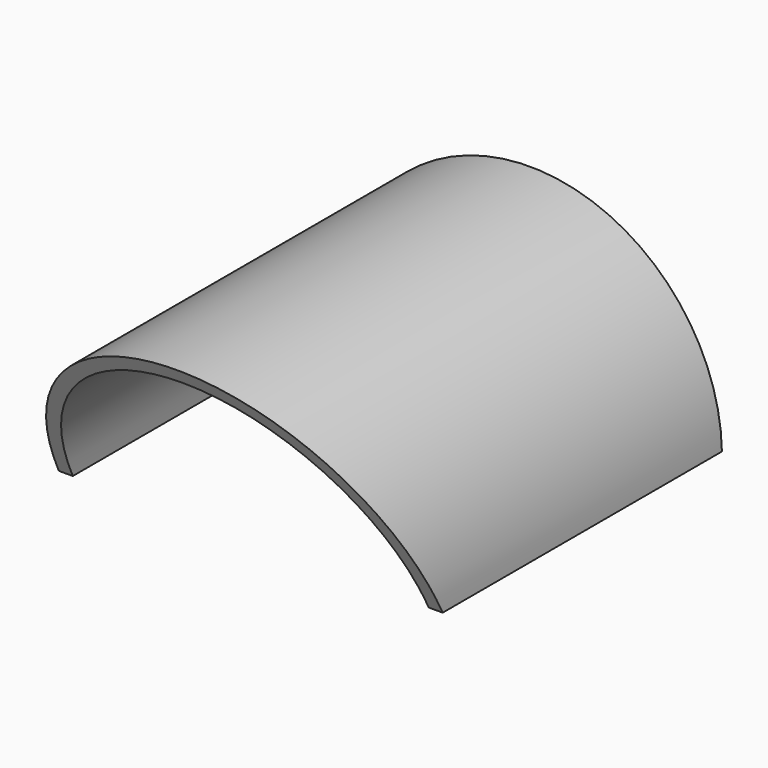
from build123d import *

# Parameters (mm, degrees)
F1_DEPTH = 127
F5_REACH = 149.52346714


with BuildPart() as f1:
    # F0 (on Front) → F1 (new body)
    with BuildSketch(Plane.XZ):
        with BuildLine():
            Line((50.9901951359, 1), (54.9909083395, 1))
            ThreePointArc((54.9909083395, 1), (0, 55), (-54.9909083395, 1))
            Line((-54.9909083395, 1), (-50.9901951359, 1))
            ThreePointArc((-50.9901951359, 1), (0, 51), (50.9901951359, 1))
        make_face()
    extrude(amount=F1_DEPTH)

    f5_end = Plane(origin=(0, -80.3890683895, -39.208368418), x_dir=(0, -0.4383711468, 0.8987940463), z_dir=(0, 0.8987940463, 0.4383711468))
    # F1_face (on face) → F5 (cut, up to a plane its end follows)
    with BuildSketch(Plane(origin=(0, -127, 34.1612155921), x_dir=(1, 0, 0), z_dir=(0, -1, 0))):
        with BuildLine():
            Line((50.9901951359, -33.1612155921), (54.9909083395, -33.1612155921))
            ThreePointArc((54.9909083395, -33.1612155921), (0, 20.8387844079), (-54.9909083395, -33.1612155921))
            Line((-54.9909083395, -33.1612155921), (-50.9901951359, -33.1612155921))
            ThreePointArc((-50.9901951359, -33.1612155921), (0, 16.8387844079), (50.9901951359, -33.1612155921))
        make_face()
    f5_long = extrude(amount=-F5_REACH, mode=Mode.PRIVATE)
    add(split(f5_long, bisect_by=f5_end, keep=Keep.BOTTOM, mode=Mode.PRIVATE), mode=Mode.SUBTRACT)


solid = f1.part
